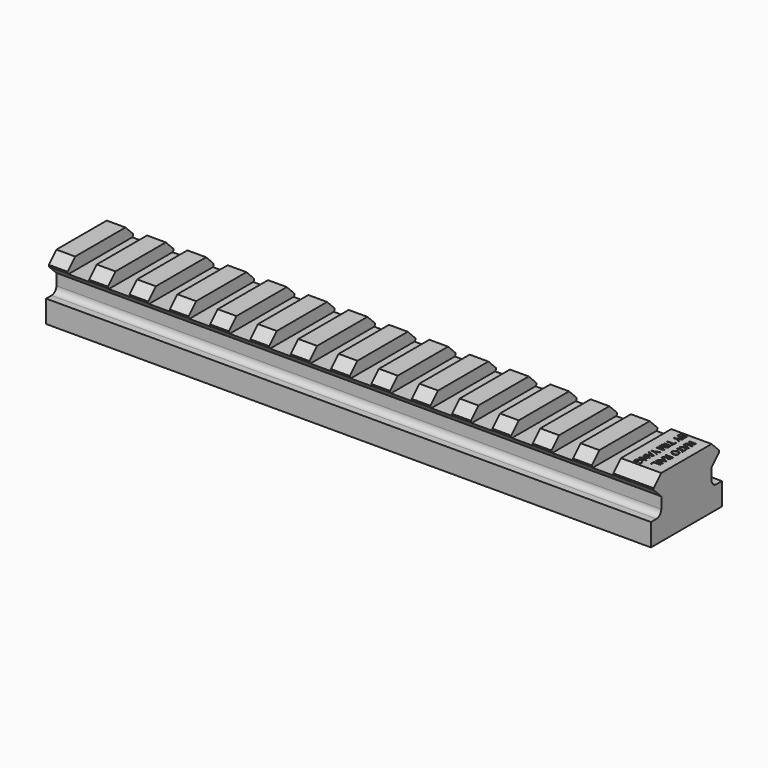
from build123d import *

# Parameters (mm, degrees)
F1_DEPTH     = 75
F2_W         = 5.35
F2_H         = 20.32
F3_DEPTH     = 3
F4_TEXT_SIZE = 2.447418738
F5_DEPTH     = 0.125


# Not quite as in the source:
# - Text() gives the source's letters only with a copy of the font that has no kerning and outlines rounded to 1/6400 em; it was checked with that copy


with BuildPart() as f1:
    # F0 (on Right) → F1 (new body, symmetric)
    with BuildSketch(Plane.YZ):
        with BuildLine():
            Line((7.8, 5.3401220269), (-7.8, 5.3401220269))
            Line((-7.8, 5.3401220269), (-10.16, 2.9801220269))
            Line((-10.16, 2.9801220269), (-10.16, 2.6001220269))
            Line((-10.16, 2.6001220269), (-7.8, 0.2401220269))
            Line((-7.8, 0.2401220269), (-7.8, -2.5598779731))
            ThreePointArc((-7.8, -2.5598779731), (-8.2393398282, -3.6205381448), (-9.3, -4.0598779731))
            Line((-9.3, -4.0598779731), (-11, -4.0598779731))
            Line((-11, -4.0598779731), (-11, -9.6106562486))
            Line((-11, -9.6106562486), (11, -9.6106562486))
            Line((11, -9.6106562486), (11, -4.0598779731))
            Line((11, -4.0598779731), (9.3, -4.0598779731))
            ThreePointArc((9.3, -4.0598779731), (8.2393398282, -3.6205381448), (7.8, -2.5598779731))
            Line((7.8, -2.5598779731), (7.8, 0.2401220269))
            Line((7.8, 0.2401220269), (10.16, 2.6001220269))
            Line((10.16, 2.6001220269), (10.16, 2.9801220269))
            Line((10.16, 2.9801220269), (7.8, 5.3401220269))
        make_face()
    extrude(amount=F1_DEPTH, both=True)

    # F2 (on face) → F3 (cut)
    with BuildSketch(Plane.XY.offset(5.3401220269)):
        with Locations((-67.675, 0)):
            Rectangle(F2_W, F2_H)
        with Locations((-57.675, 0)):
            Rectangle(F2_W, F2_H)
        with Locations((-47.675, 0)):
            Rectangle(F2_W, F2_H)
        with Locations((-37.675, 0)):
            Rectangle(F2_W, F2_H)
        with Locations((-27.675, 0)):
            Rectangle(F2_W, F2_H)
        with Locations((-17.675, 0)):
            Rectangle(F2_W, F2_H)
        with Locations((-7.675, 0)):
            Rectangle(F2_W, F2_H)
        with Locations((2.325, 0)):
            Rectangle(F2_W, F2_H)
        with Locations((12.325, 0)):
            Rectangle(F2_W, F2_H)
        with Locations((22.325, 0)):
            Rectangle(F2_W, F2_H)
        with Locations((32.325, 0)):
            Rectangle(F2_W, F2_H)
        with Locations((42.325, 0)):
            Rectangle(F2_W, F2_H)
        with Locations((52.325, 0)):
            Rectangle(F2_W, F2_H)
        with Locations((62.325, 0)):
            Rectangle(F2_W, F2_H)
    extrude(amount=-F3_DEPTH, mode=Mode.SUBTRACT)

    # F4 (on face) → F5 (cut)
    with BuildSketch(Plane.XY.offset(5.3401220269)):
        with Locations(Location((70.9878585086, 6.2281070746), (0, 0, -90))):
            Text('NATO RAIL', F4_TEXT_SIZE, font='Open Sans', text_align=(TextAlign.LEFT, TextAlign.BOTTOM))
        with Locations(Location((67.6593690249, 7.5), (0, 0, -90))):
            Text('BY TIM YANG', F4_TEXT_SIZE, font='Open Sans', text_align=(TextAlign.LEFT, TextAlign.BOTTOM))
    extrude(amount=-F5_DEPTH, mode=Mode.SUBTRACT)


solid = f1.part
